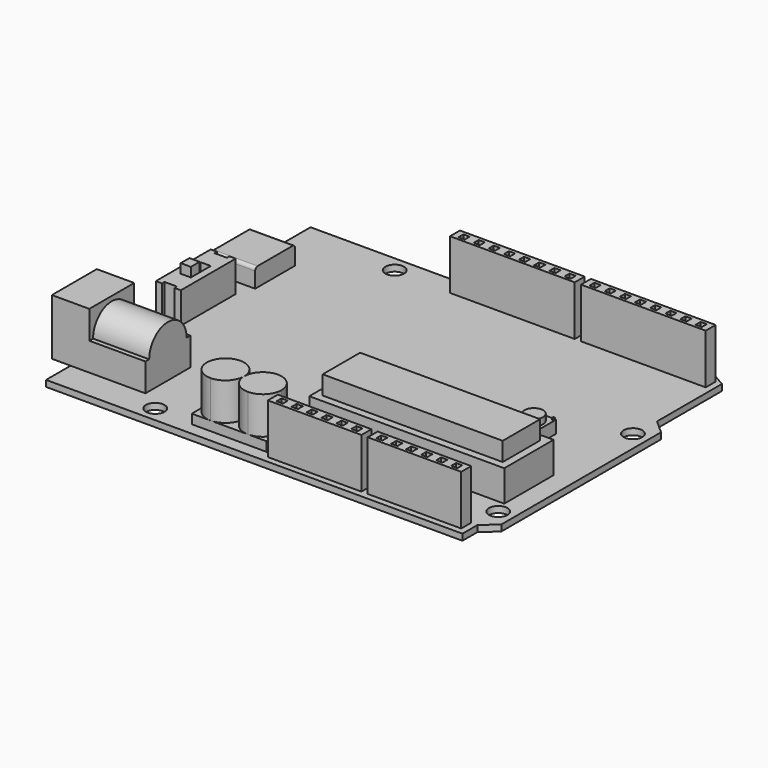
from build123d import *

# Parameters (mm, degrees)
F0_W           = 20
F0_H           = 2
F0_W_2         = 1
F0_H_2         = 1
F1_DEPTH       = 8
F0_W_3         = 15
F0_R           = 1.5
F0_W_4         = 31.2639660113
F0_H_3         = 9.8738052929
F0_W_5         = 28.8647065315
F0_H_4         = 7.49940727
F0_R_2         = 0.2
F0_W_6         = 1.6238838434
F0_H_5         = 2.25
F0_H_6         = 1.75
F0_R_3         = 0.02
F2_DEPTH       = 1
F3_DEPTH       = 5
F4_DEPTH       = 3.5
F5_DEPTH       = 6.5
F6_TEXT_SIZE   = 5.7661711859
F7_DEPTH       = 0.1
F8_DEPTH       = 1.5
F9_DEPTH       = 7.5
F10_DEPTH      = 5
F11_DEPTH      = 2
F12_DEPTH      = 3
F13_DEPTH      = 2.25
F14_W          = 9
F14_H          = 0.5
F15_DEPTH      = 12
F16_DEPTH      = 3
F17_DEPTH      = 3
F18_DEPTH      = 12
F19_DEPTH      = 12
F19_DEPTH_BACK = 3
F20_DEPTH      = 11
F20_DEPTH_BACK = 3
F21_DEPTH      = 11
F21_DEPTH_BACK = 2
F14_W_2        = 8
F14_H_2        = 3
F14_W_3        = 7.5
F14_H_3        = 2.5
F22_DEPTH      = 5
F22_DEPTH_BACK = 2
F23_R          = 0.5
F24_DEPTH      = 4.5
F24_DEPTH_BACK = 3.001
F25_DEPTH      = 8


# Not quite as in the source:
# - Text() gives the source's letters only with a copy of the font that has no kerning and outlines rounded to 1/6400 em; it was checked with that copy


with BuildPart() as f1:
    # F0 (on Top) → F1 (new body)
    with BuildSketch(Plane.XY):
        with Locations((21.2639660113, 24.5)):
            Rectangle(F0_W, F0_H)
        with Locations((12.7639660113, 24.4691212773)):
            Rectangle(F0_W_2, F0_H_2, mode=Mode.SUBTRACT)
        with Locations((15.1925374398, 24.4691212773)):
            Rectangle(F0_W_2, F0_H_2, mode=Mode.SUBTRACT)
        with Locations((17.6211088684, 24.4691212773)):
            Rectangle(F0_W_2, F0_H_2, mode=Mode.SUBTRACT)
        with Locations((20.049680297, 24.4691212773)):
            Rectangle(F0_W_2, F0_H_2, mode=Mode.SUBTRACT)
        with Locations((22.4782517255, 24.4691212773)):
            Rectangle(F0_W_2, F0_H_2, mode=Mode.SUBTRACT)
        with Locations((24.9068231541, 24.4691212773)):
            Rectangle(F0_W_2, F0_H_2, mode=Mode.SUBTRACT)
        with Locations((27.3353945827, 24.4691212773)):
            Rectangle(F0_W_2, F0_H_2, mode=Mode.SUBTRACT)
        with Locations((29.7639660113, 24.4691212773)):
            Rectangle(F0_W_2, F0_H_2, mode=Mode.SUBTRACT)
    extrude(amount=F1_DEPTH)


with BuildPart() as f1b:
    # F0 (on Top) → F1, piece 2 (new body)
    with BuildSketch(Plane.XY):
        with Locations((0.2639660113, 24.5)):
            Rectangle(F0_W, F0_H)
        with Locations((-8.2360339887, 24.4466484636)):
            Rectangle(F0_W_2, F0_H_2, mode=Mode.SUBTRACT)
        with Locations((-5.8074625602, 24.4466484636)):
            Rectangle(F0_W_2, F0_H_2, mode=Mode.SUBTRACT)
        with Locations((-3.3788911316, 24.4466484636)):
            Rectangle(F0_W_2, F0_H_2, mode=Mode.SUBTRACT)
        with Locations((-0.950319703, 24.4466484636)):
            Rectangle(F0_W_2, F0_H_2, mode=Mode.SUBTRACT)
        with Locations((1.4782517255, 24.4466484636)):
            Rectangle(F0_W_2, F0_H_2, mode=Mode.SUBTRACT)
        with Locations((3.9068231541, 24.4466484636)):
            Rectangle(F0_W_2, F0_H_2, mode=Mode.SUBTRACT)
        with Locations((6.3353945827, 24.4466484636)):
            Rectangle(F0_W_2, F0_H_2, mode=Mode.SUBTRACT)
        with Locations((8.7639660113, 24.4466484636)):
            Rectangle(F0_W_2, F0_H_2, mode=Mode.SUBTRACT)
    extrude(amount=F1_DEPTH)


with BuildPart() as f1c:
    # F0 (on Top) → F1, piece 3 (new body)
    with BuildSketch(Plane.XY):
        with Locations((23.7639660113, -24.5)):
            Rectangle(F0_W_3, F0_H)
        with Locations((17.7639660113, -24.5294059515)):
            Rectangle(F0_W_2, F0_H_2, mode=Mode.SUBTRACT)
        with Locations((20.1639660113, -24.5294059515)):
            Rectangle(F0_W_2, F0_H_2, mode=Mode.SUBTRACT)
        with Locations((22.5639660113, -24.5294059515)):
            Rectangle(F0_W_2, F0_H_2, mode=Mode.SUBTRACT)
        with Locations((24.9639660113, -24.5294059515)):
            Rectangle(F0_W_2, F0_H_2, mode=Mode.SUBTRACT)
        with Locations((27.3639660113, -24.5294059515)):
            Rectangle(F0_W_2, F0_H_2, mode=Mode.SUBTRACT)
        with Locations((29.7639660113, -24.5294059515)):
            Rectangle(F0_W_2, F0_H_2, mode=Mode.SUBTRACT)
    extrude(amount=F1_DEPTH)


with BuildPart() as f1d:
    # F0 (on Top) → F1, piece 4 (new body)
    with BuildSketch(Plane.XY):
        with Locations((7.7639660113, -24.5)):
            Rectangle(F0_W_3, F0_H)
        with Locations((1.7639660113, -24.50011383)):
            Rectangle(F0_W_2, F0_H_2, mode=Mode.SUBTRACT)
        with Locations((4.1639660113, -24.5041792203)):
            Rectangle(F0_W_2, F0_H_2, mode=Mode.SUBTRACT)
        with Locations((6.5639660113, -24.5082446107)):
            Rectangle(F0_W_2, F0_H_2, mode=Mode.SUBTRACT)
        with Locations((8.9639660113, -24.512310001)):
            Rectangle(F0_W_2, F0_H_2, mode=Mode.SUBTRACT)
        with Locations((11.3639660113, -24.5163753914)):
            Rectangle(F0_W_2, F0_H_2, mode=Mode.SUBTRACT)
        with Locations((13.7639660113, -24.5204407817)):
            Rectangle(F0_W_2, F0_H_2, mode=Mode.SUBTRACT)
    extrude(amount=F1_DEPTH)


with BuildPart() as f2:
    # F0 (on Top) → F2 (new body)
    with BuildSketch(Plane.XY):
        Polygon((32.2639660113, 25.5), (30.5319152037, 26.5), (-34.5000339887, 26.5), (-34.5000339887, 6.5), (-33.5000339887, 6.5), (-33.5000339887, 6), (-31.5000339887, 6), (-31.5000339887, 6.5), (-30.5000339887, 6.5), (-30.5000339887, -4.5), (-31.5000339887, -4.5), (-31.5000339887, -4), (-33.5000339887, -4), (-33.5000339887, -4.5), (-34.5000339887, -4.5), (-34.5000339887, -26.5), (32.2639660113, -26.5), (32.2639660113, -25.5), (32.2639660113, -23.5), (34.5000339887, -21.5), (34.5000339887, 10.5), (32.2639660113, 12.5), (32.2639660113, 23.5), align=None)
        with Locations((-19.0000339887, -24)):
            Circle(F0_R, mode=Mode.SUBTRACT)
        Polygon((-0.7360339887, -21.5), (-0.7360339887, -24.5), (-3.7360339887, -24.5), (-6.7360339887, -24.5), (-9.7360339888, -24.5), (-12.7360339887, -24.5), (-12.7360339887, -21.5), (-12.7360339887, -18.5), (-9.7360339888, -18.5), (-6.7360339887, -18.5), (-3.7360339887, -18.5), (-0.7360339887, -18.5), align=None, mode=Mode.SUBTRACT)
        with Locations((7.7639660113, -24.5)):
            Rectangle(F0_W_3, F0_H, mode=Mode.SUBTRACT)
        with Locations((23.7639660113, -24.5)):
            Rectangle(F0_W_3, F0_H, mode=Mode.SUBTRACT)
        with Locations((32.0000339887, -19)):
            Circle(F0_R, mode=Mode.SUBTRACT)
        with Locations((15.6319830056, -11.9369026465)):
            Rectangle(F0_W_4, F0_H_3, mode=Mode.SUBTRACT)
        with Locations((-19.0000339887, 24)):
            Circle(F0_R, mode=Mode.SUBTRACT)
        Polygon((20.5000339887, 1.5), (20.5000339887, 2), (21.0000339887, 2), (23.5000339887, 2), (24.0000339887, 2), (24.5000339887, 2), (24.5000339887, 1.5), (24.5000339887, 1), (24.5000339887, -1), (24.5000339887, -1.5), (24.5000339887, -2), (24.0000339887, -2), (23.5000339887, -2), (21.5000339887, -2), (21.0000339887, -2), (20.5000339887, -2), (20.5000339887, -1.5), (20.5000339887, -1), align=None, mode=Mode.SUBTRACT)
        with Locations((32.0000339887, 8)):
            Circle(F0_R, mode=Mode.SUBTRACT)
        with Locations((0.2639660113, 24.5)):
            Rectangle(F0_W, F0_H, mode=Mode.SUBTRACT)
        with Locations((21.2639660113, 24.5)):
            Rectangle(F0_W, F0_H, mode=Mode.SUBTRACT)
        with Locations((15.6319830056, -11.9369026465)):
            Rectangle(F0_W_4, F0_H_3)
        with Locations((15.6319830056, -11.9369026465)):
            Rectangle(F0_W_5, F0_H_4, mode=Mode.SUBTRACT)
        with Locations((15.6319830056, -11.9369026465)):
            Rectangle(F0_W_5, F0_H_4)
        Polygon((-33.5000339887, 6.5), (-34.5000339887, 6.5), (-34.5000339887, -4.5), (-33.5000339887, -4.5), (-33.5000339887, -4), (-31.5000339887, -4), (-31.5000339887, -4.5), (-30.5000339887, -4.5), (-30.5000339887, 6.5), (-31.5000339887, 6.5), (-31.5000339887, 6), (-33.5000339887, 6), align=None)
        Polygon((-33.3119759105, 0.75), (-33.3119759105, 3), (-31.688092067, 3), (-31.688092067, 0.75), (-31.688092067, -1), (-33.3119759105, -1), align=None, mode=Mode.SUBTRACT)
        with Locations((0.2639660113, 24.5)):
            Rectangle(F0_W, F0_H)
        with Locations((-8.2360339887, 24.4466484636)):
            Rectangle(F0_W_2, F0_H_2, mode=Mode.SUBTRACT)
        with Locations((-5.8074625602, 24.4466484636)):
            Rectangle(F0_W_2, F0_H_2, mode=Mode.SUBTRACT)
        with Locations((-3.3788911316, 24.4466484636)):
            Rectangle(F0_W_2, F0_H_2, mode=Mode.SUBTRACT)
        with Locations((-0.950319703, 24.4466484636)):
            Rectangle(F0_W_2, F0_H_2, mode=Mode.SUBTRACT)
        with Locations((1.4782517255, 24.4466484636)):
            Rectangle(F0_W_2, F0_H_2, mode=Mode.SUBTRACT)
        with Locations((3.9068231541, 24.4466484636)):
            Rectangle(F0_W_2, F0_H_2, mode=Mode.SUBTRACT)
        with Locations((6.3353945827, 24.4466484636)):
            Rectangle(F0_W_2, F0_H_2, mode=Mode.SUBTRACT)
        with Locations((8.7639660113, 24.4466484636)):
            Rectangle(F0_W_2, F0_H_2, mode=Mode.SUBTRACT)
        with Locations((21.2639660113, 24.5)):
            Rectangle(F0_W, F0_H)
        with Locations((12.7639660113, 24.4691212773)):
            Rectangle(F0_W_2, F0_H_2, mode=Mode.SUBTRACT)
        with Locations((15.1925374398, 24.4691212773)):
            Rectangle(F0_W_2, F0_H_2, mode=Mode.SUBTRACT)
        with Locations((17.6211088684, 24.4691212773)):
            Rectangle(F0_W_2, F0_H_2, mode=Mode.SUBTRACT)
        with Locations((20.049680297, 24.4691212773)):
            Rectangle(F0_W_2, F0_H_2, mode=Mode.SUBTRACT)
        with Locations((22.4782517255, 24.4691212773)):
            Rectangle(F0_W_2, F0_H_2, mode=Mode.SUBTRACT)
        with Locations((24.9068231541, 24.4691212773)):
            Rectangle(F0_W_2, F0_H_2, mode=Mode.SUBTRACT)
        with Locations((27.3353945827, 24.4691212773)):
            Rectangle(F0_W_2, F0_H_2, mode=Mode.SUBTRACT)
        with Locations((29.7639660113, 24.4691212773)):
            Rectangle(F0_W_2, F0_H_2, mode=Mode.SUBTRACT)
        with Locations((7.7639660113, -24.5)):
            Rectangle(F0_W_3, F0_H)
        with Locations((1.7639660113, -24.50011383)):
            Rectangle(F0_W_2, F0_H_2, mode=Mode.SUBTRACT)
        with Locations((4.1639660113, -24.5041792203)):
            Rectangle(F0_W_2, F0_H_2, mode=Mode.SUBTRACT)
        with Locations((6.5639660113, -24.5082446107)):
            Rectangle(F0_W_2, F0_H_2, mode=Mode.SUBTRACT)
        with Locations((8.9639660113, -24.512310001)):
            Rectangle(F0_W_2, F0_H_2, mode=Mode.SUBTRACT)
        with Locations((11.3639660113, -24.5163753914)):
            Rectangle(F0_W_2, F0_H_2, mode=Mode.SUBTRACT)
        with Locations((13.7639660113, -24.5204407817)):
            Rectangle(F0_W_2, F0_H_2, mode=Mode.SUBTRACT)
        with Locations((23.7639660113, -24.5)):
            Rectangle(F0_W_3, F0_H)
        with Locations((17.7639660113, -24.5294059515)):
            Rectangle(F0_W_2, F0_H_2, mode=Mode.SUBTRACT)
        with Locations((20.1639660113, -24.5294059515)):
            Rectangle(F0_W_2, F0_H_2, mode=Mode.SUBTRACT)
        with Locations((22.5639660113, -24.5294059515)):
            Rectangle(F0_W_2, F0_H_2, mode=Mode.SUBTRACT)
        with Locations((24.9639660113, -24.5294059515)):
            Rectangle(F0_W_2, F0_H_2, mode=Mode.SUBTRACT)
        with Locations((27.3639660113, -24.5294059515)):
            Rectangle(F0_W_2, F0_H_2, mode=Mode.SUBTRACT)
        with Locations((29.7639660113, -24.5294059515)):
            Rectangle(F0_W_2, F0_H_2, mode=Mode.SUBTRACT)
        with BuildLine():
            ThreePointArc((-6.7360339887, -21.5), (-5.8573543323, -23.6213203436), (-3.7360339887, -24.5))
            ThreePointArc((-3.7360339887, -24.5), (-1.6147136452, -23.6213203436), (-0.7360339887, -21.5))
            ThreePointArc((-0.7360339887, -21.5), (-1.6147136452, -19.3786796564), (-3.7360339887, -18.5))
            ThreePointArc((-3.7360339887, -18.5), (-5.8573543323, -19.3786796564), (-6.7360339887, -21.5))
        make_face()
        with BuildLine():
            ThreePointArc((-9.7360339888, -24.5), (-7.6147136452, -23.6213203436), (-6.7360339887, -21.5))
            ThreePointArc((-6.7360339887, -21.5), (-7.6147136452, -19.3786796564), (-9.7360339888, -18.5))
            ThreePointArc((-9.7360339888, -18.5), (-11.8573543323, -19.3786796564), (-12.7360339887, -21.5))
            ThreePointArc((-12.7360339887, -21.5), (-11.8573543323, -23.6213203436), (-9.7360339888, -24.5))
        make_face()
        Polygon((21.0000339887, 2), (20.5000339887, 2), (20.5000339887, 1.5), (20.5000339887, -1), (20.5000339887, -1.5), (20.5000339887, -2), (21.0000339887, -2), (21.5000339887, -2), (23.5000339887, -2), (24.0000339887, -2), (24.5000339887, -2), (24.5000339887, -1.5), (24.5000339887, -1), (24.5000339887, 1), (24.5000339887, 1.5), (24.5000339887, 2), (24.0000339887, 2), (23.5000339887, 2), align=None)
        with Locations((20.7500339887, -1.75)):
            Circle(F0_R_2, mode=Mode.SUBTRACT)
        with Locations((24.2500339887, -1.75)):
            Circle(F0_R_2, mode=Mode.SUBTRACT)
        with Locations((20.7500339887, 1.75)):
            Circle(F0_R_2, mode=Mode.SUBTRACT)
        with Locations((22.5000339887, 0)):
            Circle(F0_R, mode=Mode.SUBTRACT)
        with Locations((24.2500339887, 1.75)):
            Circle(F0_R_2, mode=Mode.SUBTRACT)
        with Locations((22.5000339887, 0)):
            Circle(F0_R)
        with Locations((-32.5000339887, 1.875)):
            Rectangle(F0_W_6, F0_H_5)
        with Locations((-32.5000339887, -0.125)):
            Rectangle(F0_W_6, F0_H_6)
        with BuildLine():
            Line((-6.7360339887, -18.5), (-6.7360339887, -21.5))
            ThreePointArc((-6.7360339887, -21.5), (-5.8573543323, -19.3786796564), (-3.7360339887, -18.5))
            Line((-3.7360339887, -18.5), (-6.7360339887, -18.5))
        make_face()
        with BuildLine():
            ThreePointArc((-3.7360339887, -18.5), (-1.6147136452, -19.3786796564), (-0.7360339887, -21.5))
            Line((-0.7360339887, -21.5), (-0.7360339887, -18.5))
            Line((-0.7360339887, -18.5), (-3.7360339887, -18.5))
        make_face()
        with BuildLine():
            Line((-6.7360339887, -24.5), (-3.7360339887, -24.5))
            ThreePointArc((-3.7360339887, -24.5), (-5.8573543323, -23.6213203436), (-6.7360339887, -21.5))
            Line((-6.7360339887, -21.5), (-6.7360339887, -24.5))
        make_face()
        with BuildLine():
            Line((-3.7360339887, -24.5), (-0.7360339887, -24.5))
            Line((-0.7360339887, -24.5), (-0.7360339887, -21.5))
            ThreePointArc((-0.7360339887, -21.5), (-1.6147136452, -23.6213203436), (-3.7360339887, -24.5))
        make_face()
        with BuildLine():
            Line((-9.7360339888, -24.5), (-6.7360339887, -24.5))
            Line((-6.7360339887, -24.5), (-6.7360339887, -21.5))
            ThreePointArc((-6.7360339887, -21.5), (-7.6147136452, -23.6213203436), (-9.7360339888, -24.5))
        make_face()
        with BuildLine():
            Line((-12.7360339887, -24.5), (-9.7360339888, -24.5))
            ThreePointArc((-9.7360339888, -24.5), (-11.8573543323, -23.6213203436), (-12.7360339887, -21.5))
            Line((-12.7360339887, -21.5), (-12.7360339887, -24.5))
        make_face()
        with BuildLine():
            ThreePointArc((-12.7360339887, -21.5), (-11.8573543323, -19.3786796564), (-9.7360339888, -18.5))
            Line((-9.7360339888, -18.5), (-12.7360339887, -18.5))
            Line((-12.7360339887, -18.5), (-12.7360339887, -21.5))
        make_face()
        with BuildLine():
            ThreePointArc((-9.7360339888, -18.5), (-7.6147136452, -19.3786796564), (-6.7360339887, -21.5))
            Line((-6.7360339887, -21.5), (-6.7360339887, -18.5))
            Line((-6.7360339887, -18.5), (-9.7360339888, -18.5))
        make_face()
        with Locations((8.9639660113, -24.512310001)):
            Rectangle(F0_W_2, F0_H_2)
        with Locations((11.3639660113, -24.5163753914)):
            Rectangle(F0_W_2, F0_H_2)
        with Locations((13.7639660113, -24.5204407817)):
            Rectangle(F0_W_2, F0_H_2)
        with Locations((17.7639660113, -24.5294059515)):
            Rectangle(F0_W_2, F0_H_2)
        with Locations((20.1639660113, -24.5294059515)):
            Rectangle(F0_W_2, F0_H_2)
        with Locations((22.5639660113, -24.5294059515)):
            Rectangle(F0_W_2, F0_H_2)
        with Locations((27.3639660113, -24.5294059515)):
            Rectangle(F0_W_2, F0_H_2)
        with Locations((29.7639660113, -24.5294059515)):
            Rectangle(F0_W_2, F0_H_2)
        with Locations((24.9639660113, -24.5294059515)):
            Rectangle(F0_W_2, F0_H_2)
        with Locations((-8.2360339887, 24.4466484636)):
            Rectangle(F0_W_2, F0_H_2)
        with Locations((-5.8074625602, 24.4466484636)):
            Rectangle(F0_W_2, F0_H_2)
        with Locations((-3.3788911316, 24.4466484636)):
            Rectangle(F0_W_2, F0_H_2)
        with Locations((-0.950319703, 24.4466484636)):
            Rectangle(F0_W_2, F0_H_2)
        with Locations((1.4782517255, 24.4466484636)):
            Rectangle(F0_W_2, F0_H_2)
        with Locations((3.9068231541, 24.4466484636)):
            Rectangle(F0_W_2, F0_H_2)
        with Locations((6.3353945827, 24.4466484636)):
            Rectangle(F0_W_2, F0_H_2)
        with Locations((8.7639660113, 24.4466484636)):
            Rectangle(F0_W_2, F0_H_2)
        with Locations((12.7639660113, 24.4691212773)):
            Rectangle(F0_W_2, F0_H_2)
        with Locations((17.6211088684, 24.4691212773)):
            Rectangle(F0_W_2, F0_H_2)
        with Locations((20.049680297, 24.4691212773)):
            Rectangle(F0_W_2, F0_H_2)
        with Locations((22.4782517255, 24.4691212773)):
            Rectangle(F0_W_2, F0_H_2)
        with Locations((24.9068231541, 24.4691212773)):
            Rectangle(F0_W_2, F0_H_2)
        with Locations((27.3353945827, 24.4691212773)):
            Rectangle(F0_W_2, F0_H_2)
        with Locations((29.7639660113, 24.4691212773)):
            Rectangle(F0_W_2, F0_H_2)
        with Locations((15.1925374398, 24.4691212773)):
            Rectangle(F0_W_2, F0_H_2)
        with Locations((1.7639660113, -24.50011383)):
            Rectangle(F0_W_2, F0_H_2)
        with Locations((4.1639660113, -24.5041792203)):
            Rectangle(F0_W_2, F0_H_2)
        with Locations((6.5639660113, -24.5082446107)):
            Rectangle(F0_W_2, F0_H_2)
        with Locations((20.7500339887, -1.75)):
            Circle(F0_R_2)
        with Locations((20.7500339887, -1.75)):
            Circle(F0_R_3, mode=Mode.SUBTRACT)
        with Locations((24.2500339887, -1.75)):
            Circle(F0_R_2)
        with Locations((24.2500339887, 1.75)):
            Circle(F0_R_2)
        with Locations((20.7500339887, 1.75)):
            Circle(F0_R_2)
    extrude(amount=-F2_DEPTH)

    # F6 (on face) → F7 (cut)
    with BuildSketch(Plane(origin=(0, 0, -1), x_dir=(1, 0, 0), z_dir=(0, 0, -1))):
        with Locations((-31.5797924995, 10.7959639281)):
            Text('Michael Ma', F6_TEXT_SIZE, font='Open Sans', text_align=(TextAlign.LEFT, TextAlign.BOTTOM))
        with Locations((-31.5797924995, 2.9539711153)):
            Text('Derek Ni', F6_TEXT_SIZE, font='Open Sans', text_align=(TextAlign.LEFT, TextAlign.BOTTOM))
    extrude(amount=-F7_DEPTH, mode=Mode.SUBTRACT)


with BuildPart() as f3:
    # F0 (on Top) → F3 (new body)
    with BuildSketch(Plane.XY):
        Polygon((-33.5000339887, 6.5), (-34.5000339887, 6.5), (-34.5000339887, -4.5), (-33.5000339887, -4.5), (-33.5000339887, -4), (-31.5000339887, -4), (-31.5000339887, -4.5), (-30.5000339887, -4.5), (-30.5000339887, 6.5), (-31.5000339887, 6.5), (-31.5000339887, 6), (-33.5000339887, 6), align=None)
        Polygon((-33.3119759105, 0.75), (-33.3119759105, 3), (-31.688092067, 3), (-31.688092067, 0.75), (-31.688092067, -1), (-33.3119759105, -1), align=None, mode=Mode.SUBTRACT)
    extrude(amount=F3_DEPTH)


with BuildPart() as f4:
    # F0 (on Top) → F4 (new body)
    with BuildSketch(Plane.XY):
        with Locations((-32.5000339887, 1.875)):
            Rectangle(F0_W_6, F0_H_5)
        with Locations((-32.5000339887, -0.125)):
            Rectangle(F0_W_6, F0_H_6)
    extrude(amount=F4_DEPTH)


with BuildPart() as f5:
    # F0 (on Top) → F5 (new body)
    with BuildSketch(Plane.XY):
        with Locations((-32.5000339887, -0.125)):
            Rectangle(F0_W_6, F0_H_6)
    extrude(amount=F5_DEPTH)


with BuildPart() as f8:
    # F0 (on Top) → F8 (new body)
    with BuildSketch(Plane.XY):
        with BuildLine():
            ThreePointArc((-9.7360339888, -18.5), (-7.6147136452, -19.3786796564), (-6.7360339887, -21.5))
            Line((-6.7360339887, -21.5), (-6.7360339887, -18.5))
            Line((-6.7360339887, -18.5), (-9.7360339888, -18.5))
        make_face()
        with BuildLine():
            ThreePointArc((-12.7360339887, -21.5), (-11.8573543323, -19.3786796564), (-9.7360339888, -18.5))
            Line((-9.7360339888, -18.5), (-12.7360339887, -18.5))
            Line((-12.7360339887, -18.5), (-12.7360339887, -21.5))
        make_face()
        with BuildLine():
            Line((-12.7360339887, -24.5), (-9.7360339888, -24.5))
            ThreePointArc((-9.7360339888, -24.5), (-11.8573543323, -23.6213203436), (-12.7360339887, -21.5))
            Line((-12.7360339887, -21.5), (-12.7360339887, -24.5))
        make_face()
        with BuildLine():
            Line((-9.7360339888, -24.5), (-6.7360339887, -24.5))
            Line((-6.7360339887, -24.5), (-6.7360339887, -21.5))
            ThreePointArc((-6.7360339887, -21.5), (-7.6147136452, -23.6213203436), (-9.7360339888, -24.5))
        make_face()
        with BuildLine():
            ThreePointArc((-9.7360339888, -24.5), (-7.6147136452, -23.6213203436), (-6.7360339887, -21.5))
            ThreePointArc((-6.7360339887, -21.5), (-7.6147136452, -19.3786796564), (-9.7360339888, -18.5))
            ThreePointArc((-9.7360339888, -18.5), (-11.8573543323, -19.3786796564), (-12.7360339887, -21.5))
            ThreePointArc((-12.7360339887, -21.5), (-11.8573543323, -23.6213203436), (-9.7360339888, -24.5))
        make_face()
        with BuildLine():
            ThreePointArc((-6.7360339887, -21.5), (-5.8573543323, -23.6213203436), (-3.7360339887, -24.5))
            ThreePointArc((-3.7360339887, -24.5), (-1.6147136452, -23.6213203436), (-0.7360339887, -21.5))
            ThreePointArc((-0.7360339887, -21.5), (-1.6147136452, -19.3786796564), (-3.7360339887, -18.5))
            ThreePointArc((-3.7360339887, -18.5), (-5.8573543323, -19.3786796564), (-6.7360339887, -21.5))
        make_face()
        with BuildLine():
            Line((-6.7360339887, -18.5), (-6.7360339887, -21.5))
            ThreePointArc((-6.7360339887, -21.5), (-5.8573543323, -19.3786796564), (-3.7360339887, -18.5))
            Line((-3.7360339887, -18.5), (-6.7360339887, -18.5))
        make_face()
        with BuildLine():
            ThreePointArc((-3.7360339887, -18.5), (-1.6147136452, -19.3786796564), (-0.7360339887, -21.5))
            Line((-0.7360339887, -21.5), (-0.7360339887, -18.5))
            Line((-0.7360339887, -18.5), (-3.7360339887, -18.5))
        make_face()
        with BuildLine():
            Line((-3.7360339887, -24.5), (-0.7360339887, -24.5))
            Line((-0.7360339887, -24.5), (-0.7360339887, -21.5))
            ThreePointArc((-0.7360339887, -21.5), (-1.6147136452, -23.6213203436), (-3.7360339887, -24.5))
        make_face()
        with BuildLine():
            Line((-6.7360339887, -24.5), (-3.7360339887, -24.5))
            ThreePointArc((-3.7360339887, -24.5), (-5.8573543323, -23.6213203436), (-6.7360339887, -21.5))
            Line((-6.7360339887, -21.5), (-6.7360339887, -24.5))
        make_face()
    extrude(amount=F8_DEPTH)


with BuildPart() as f9:
    # F0 (on Top) → F9 (new body)
    with BuildSketch(Plane.XY):
        with BuildLine():
            ThreePointArc((-6.7360339887, -21.5), (-5.8573543323, -23.6213203436), (-3.7360339887, -24.5))
            ThreePointArc((-3.7360339887, -24.5), (-1.6147136452, -23.6213203436), (-0.7360339887, -21.5))
            ThreePointArc((-0.7360339887, -21.5), (-1.6147136452, -19.3786796564), (-3.7360339887, -18.5))
            ThreePointArc((-3.7360339887, -18.5), (-5.8573543323, -19.3786796564), (-6.7360339887, -21.5))
        make_face()
    extrude(amount=F9_DEPTH)


with BuildPart() as f9b:
    # F0 (on Top) → F9, piece 2 (new body)
    with BuildSketch(Plane.XY):
        with BuildLine():
            ThreePointArc((-9.7360339888, -24.5), (-7.6147136452, -23.6213203436), (-6.7360339887, -21.5))
            ThreePointArc((-6.7360339887, -21.5), (-7.6147136452, -19.3786796564), (-9.7360339888, -18.5))
            ThreePointArc((-9.7360339888, -18.5), (-11.8573543323, -19.3786796564), (-12.7360339887, -21.5))
            ThreePointArc((-12.7360339887, -21.5), (-11.8573543323, -23.6213203436), (-9.7360339888, -24.5))
        make_face()
    extrude(amount=F9_DEPTH)


with BuildPart() as f10:
    # F0 (on Top) → F10 (new body)
    with BuildSketch(Plane.XY):
        with Locations((15.6319830056, -11.9369026465)):
            Rectangle(F0_W_4, F0_H_3)
        with Locations((15.6319830056, -11.9369026465)):
            Rectangle(F0_W_5, F0_H_4, mode=Mode.SUBTRACT)
    extrude(amount=F10_DEPTH)

    # F0 (on Top) → F25 (join)
    with BuildSketch(Plane.XY):
        with Locations((15.6319830056, -11.9369026465)):
            Rectangle(F0_W_5, F0_H_4)
    extrude(amount=F25_DEPTH)


with BuildPart() as f11:
    # F0 (on Top) → F11 (new body)
    with BuildSketch(Plane.XY):
        Polygon((21.0000339887, 2), (20.5000339887, 2), (20.5000339887, 1.5), (20.5000339887, -1), (20.5000339887, -1.5), (20.5000339887, -2), (21.0000339887, -2), (21.5000339887, -2), (23.5000339887, -2), (24.0000339887, -2), (24.5000339887, -2), (24.5000339887, -1.5), (24.5000339887, -1), (24.5000339887, 1), (24.5000339887, 1.5), (24.5000339887, 2), (24.0000339887, 2), (23.5000339887, 2), align=None)
        with Locations((20.7500339887, -1.75)):
            Circle(F0_R_2, mode=Mode.SUBTRACT)
        with Locations((24.2500339887, -1.75)):
            Circle(F0_R_2, mode=Mode.SUBTRACT)
        with Locations((20.7500339887, 1.75)):
            Circle(F0_R_2, mode=Mode.SUBTRACT)
        with Locations((22.5000339887, 0)):
            Circle(F0_R, mode=Mode.SUBTRACT)
        with Locations((24.2500339887, 1.75)):
            Circle(F0_R_2, mode=Mode.SUBTRACT)
        with Locations((22.5000339887, 0)):
            Circle(F0_R)
    extrude(amount=F11_DEPTH)


with BuildPart() as f12:
    # F0 (on Top) → F12 (new body)
    with BuildSketch(Plane.XY):
        with Locations((22.5000339887, 0)):
            Circle(F0_R)
    extrude(amount=F12_DEPTH)


with BuildPart() as f13:
    # F0 (on Top) → F13 (new body)
    with BuildSketch(Plane.XY):
        with Locations((20.7500339887, 1.75)):
            Circle(F0_R_2)
    extrude(amount=F13_DEPTH)


with BuildPart() as f13b:
    # F0 (on Top) → F13, piece 2 (new body)
    with BuildSketch(Plane.XY):
        with Locations((24.2500339887, 1.75)):
            Circle(F0_R_2)
    extrude(amount=F13_DEPTH)


with BuildPart() as f13c:
    # F0 (on Top) → F13, piece 3 (new body)
    with BuildSketch(Plane.XY):
        with Locations((24.2500339887, -1.75)):
            Circle(F0_R_2)
    extrude(amount=F13_DEPTH)


with BuildPart() as f13d:
    # F0 (on Top) → F13, piece 4 (new body)
    with BuildSketch(Plane.XY):
        with Locations((20.7500339887, -1.75)):
            Circle(F0_R_2)
        with Locations((20.7500339887, -1.75)):
            Circle(F0_R_3, mode=Mode.SUBTRACT)
    extrude(amount=F13_DEPTH)


with BuildPart() as f15:
    # F14 (on face) → F15 (new body)
    with BuildSketch(Plane(origin=(-34.5000339887, 0, 0), x_dir=(0, -1, 0), z_dir=(-1, 0, 0))):
        with Locations((17.0849023461, 0.25)):
            Rectangle(F14_W, F14_H)
    extrude(amount=-F15_DEPTH)

    # F16 (add): a face of the model
    f16_faces = [f15.faces().sort_by_distance(p)[0] for p in [
        (-34.5000339887, -17.0849023461, 0.25),
    ]]
    extrude(f16_faces, amount=F16_DEPTH)

    # F14 (on face) → F17 (join, symmetric)
    with BuildSketch(Plane(origin=(-34.5000339887, 0, 0), x_dir=(0, -1, 0), z_dir=(-1, 0, 0))):
        with BuildLine():
            Line((12.5849023461, 9), (12.5849023461, 4.5))
            Line((12.5849023461, 4.5), (13.3349023461, 4.5))
            ThreePointArc((13.3349023461, 4.5), (17.0849023461, 8.25), (20.8349023461, 4.5))
            Line((20.8349023461, 4.5), (21.5849023461, 4.5))
            Line((21.5849023461, 4.5), (21.5849023461, 9))
            Line((21.5849023461, 9), (12.5849023461, 9))
        make_face()
        with BuildLine():
            Line((12.5849023461, 4.5), (12.5849023461, 0.5))
            Line((12.5849023461, 0.5), (21.5849023461, 0.5))
            Line((21.5849023461, 0.5), (21.5849023461, 4.5))
            Line((21.5849023461, 4.5), (20.8349023461, 4.5))
            ThreePointArc((20.8349023461, 4.5), (17.0849023461, 0.75), (13.3349023461, 4.5))
            Line((13.3349023461, 4.5), (12.5849023461, 4.5))
        make_face()
    extrude(amount=F17_DEPTH, both=True)

    # F14 (on face) → F18 (join)
    with BuildSketch(Plane(origin=(-34.5000339887, 0, 0), x_dir=(0, -1, 0), z_dir=(-1, 0, 0))):
        with BuildLine():
            Line((12.5849023461, 4.5), (12.5849023461, 0.5))
            Line((12.5849023461, 0.5), (21.5849023461, 0.5))
            Line((21.5849023461, 0.5), (21.5849023461, 4.5))
            Line((21.5849023461, 4.5), (20.8349023461, 4.5))
            ThreePointArc((20.8349023461, 4.5), (17.0849023461, 0.75), (13.3349023461, 4.5))
            Line((13.3349023461, 4.5), (12.5849023461, 4.5))
        make_face()
    extrude(amount=-F18_DEPTH)

    # F14 (on face) → F19 (join, two sides)
    with BuildSketch(Plane(origin=(-34.5000339887, 0, 0), x_dir=(0, -1, 0), z_dir=(-1, 0, 0))) as f19_sk:
        with BuildLine():
            Line((13.5849023461, 4.5), (13.3349023461, 4.5))
            ThreePointArc((13.3349023461, 4.5), (17.0849023461, 0.75), (20.8349023461, 4.5))
            Line((20.8349023461, 4.5), (20.5849023461, 4.5))
            ThreePointArc((20.5849023461, 4.5), (17.0849023461, 1), (13.5849023461, 4.5))
        make_face()
        with BuildLine():
            ThreePointArc((20.8349023461, 4.5), (17.0849023461, 8.25), (13.3349023461, 4.5))
            Line((13.3349023461, 4.5), (13.5849023461, 4.5))
            ThreePointArc((13.5849023461, 4.5), (17.0849023461, 8), (20.5849023461, 4.5))
            Line((20.5849023461, 4.5), (20.8349023461, 4.5))
        make_face()
        with BuildLine():
            Line((16.5849023461, 4.5), (13.5849023461, 4.5))
            ThreePointArc((13.5849023461, 4.5), (17.0849023461, 1), (20.5849023461, 4.5))
            Line((20.5849023461, 4.5), (17.5849023461, 4.5))
            ThreePointArc((17.5849023461, 4.5), (17.0849023461, 4), (16.5849023461, 4.5))
        make_face()
        with BuildLine():
            ThreePointArc((20.5849023461, 4.5), (17.0849023461, 8), (13.5849023461, 4.5))
            Line((13.5849023461, 4.5), (16.5849023461, 4.5))
            ThreePointArc((16.5849023461, 4.5), (17.0849023461, 5), (17.5849023461, 4.5))
            Line((17.5849023461, 4.5), (20.5849023461, 4.5))
        make_face()
        with BuildLine():
            Line((17.5849023461, 4.5), (16.5849023461, 4.5))
            ThreePointArc((16.5849023461, 4.5), (17.0849023461, 4), (17.5849023461, 4.5))
        make_face()
        with BuildLine():
            ThreePointArc((17.5849023461, 4.5), (17.0849023461, 5), (16.5849023461, 4.5))
            Line((16.5849023461, 4.5), (17.5849023461, 4.5))
        make_face()
    extrude(amount=-F19_DEPTH)
    extrude(f19_sk.sketch, amount=F19_DEPTH_BACK)

    # F14 (on face) → F20 (cut, two sides)
    with BuildSketch(Plane(origin=(-34.5000339887, 0, 0), x_dir=(0, -1, 0), z_dir=(-1, 0, 0))) as f20_sk:
        with BuildLine():
            Line((16.5849023461, 4.5), (13.5849023461, 4.5))
            ThreePointArc((13.5849023461, 4.5), (17.0849023461, 1), (20.5849023461, 4.5))
            Line((20.5849023461, 4.5), (17.5849023461, 4.5))
            ThreePointArc((17.5849023461, 4.5), (17.0849023461, 4), (16.5849023461, 4.5))
        make_face()
        with BuildLine():
            ThreePointArc((20.5849023461, 4.5), (17.0849023461, 8), (13.5849023461, 4.5))
            Line((13.5849023461, 4.5), (16.5849023461, 4.5))
            ThreePointArc((16.5849023461, 4.5), (17.0849023461, 5), (17.5849023461, 4.5))
            Line((17.5849023461, 4.5), (20.5849023461, 4.5))
        make_face()
        with BuildLine():
            ThreePointArc((17.5849023461, 4.5), (17.0849023461, 5), (16.5849023461, 4.5))
            Line((16.5849023461, 4.5), (17.5849023461, 4.5))
        make_face()
        with BuildLine():
            Line((17.5849023461, 4.5), (16.5849023461, 4.5))
            ThreePointArc((16.5849023461, 4.5), (17.0849023461, 4), (17.5849023461, 4.5))
        make_face()
    extrude(amount=-F20_DEPTH, mode=Mode.SUBTRACT)
    extrude(f20_sk.sketch, amount=F20_DEPTH_BACK, mode=Mode.SUBTRACT)


with BuildPart() as f21:
    # F14 (on face) → F21 (new body, two sides)
    with BuildSketch(Plane(origin=(-34.5000339887, 0, 0), x_dir=(0, -1, 0), z_dir=(-1, 0, 0))) as f21_sk:
        with BuildLine():
            Line((17.5849023461, 4.5), (16.5849023461, 4.5))
            ThreePointArc((16.5849023461, 4.5), (17.0849023461, 4), (17.5849023461, 4.5))
        make_face()
        with BuildLine():
            ThreePointArc((17.5849023461, 4.5), (17.0849023461, 5), (16.5849023461, 4.5))
            Line((16.5849023461, 4.5), (17.5849023461, 4.5))
        make_face()
    extrude(amount=-F21_DEPTH)
    extrude(f21_sk.sketch, amount=F21_DEPTH_BACK)


with BuildPart() as f22:
    # F14 (on face) → F22 (new body, two sides)
    with BuildSketch(Plane(origin=(-34.5000339887, 0, 0), x_dir=(0, -1, 0), z_dir=(-1, 0, 0))) as f22_sk:
        with Locations((-13.1479638666, 1.5)):
            Rectangle(F14_W_2, F14_H_2)
        with Locations((-13.1479638666, 1.5)):
            Rectangle(F14_W_3, F14_H_3, mode=Mode.SUBTRACT)
        with Locations((-13.1479638666, 1.5)):
            Rectangle(F14_W_3, F14_H_3)
    extrude(amount=-F22_DEPTH)
    extrude(f22_sk.sketch, amount=F22_DEPTH_BACK)

    # F23
    f23_edges = [f22.edges().sort_by_distance(p)[0] for p in [
        (-33.000034, 9.147964, 3),
        (-33.000034, 17.147964, 3),
    ]]
    fillet(f23_edges, radius=F23_R)

    # F14 (on face) → F24 (cut, two sides)
    with BuildSketch(Plane(origin=(-34.5000339887, 0, 0), x_dir=(0, -1, 0), z_dir=(-1, 0, 0))) as f24_sk:
        with Locations((-13.1479638666, 1.5)):
            Rectangle(F14_W_3, F14_H_3)
    extrude(amount=-F24_DEPTH, mode=Mode.SUBTRACT)
    extrude(f24_sk.sketch, amount=F24_DEPTH_BACK, mode=Mode.SUBTRACT)


solid = Compound([f1.part, f1b.part, f1c.part, f1d.part, f2.part, f3.part, f4.part, f5.part, f8.part, f9.part, f9b.part, f10.part, f11.part, f12.part, f13.part, f13b.part, f13c.part, f13d.part, f15.part, f21.part, f22.part])
